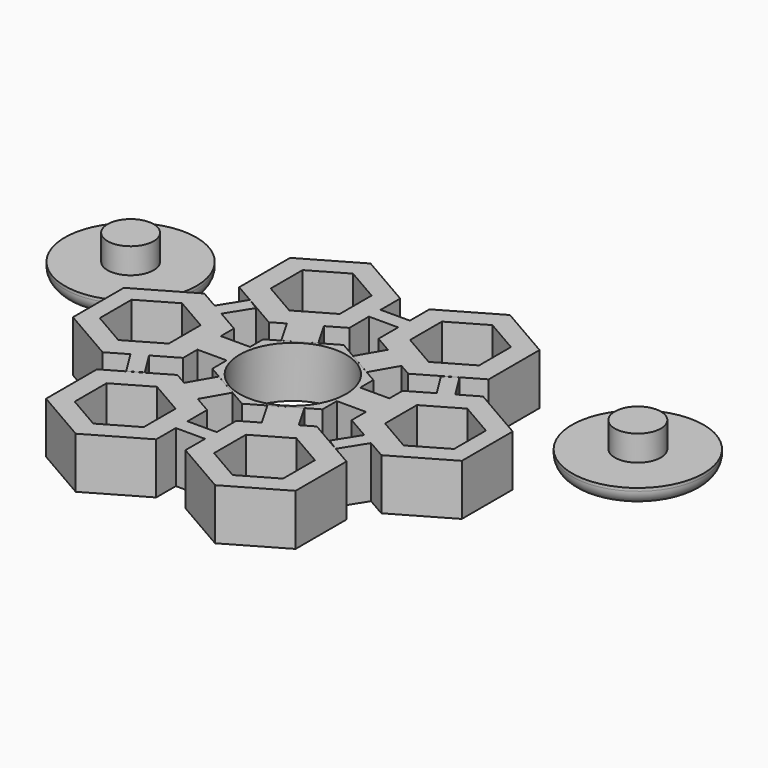
from build123d import *

# Parameters (mm, degrees)
F0_R          = 9.2578738012
F0_W          = 5.08
F0_H          = 5.08
F1_DEPTH      = 8.89
F0_H_2        = 2.54
F3_DEPTH      = 8.89
F4_R          = 11.43
F5_DEPTH      = 3.048
F6_R          = 4.0005
F7_DEPTH      = 4.445
F8_R          = 2.54
F9_TEXT_SIZE  = 11.5541534291
F10_DEPTH     = 1.524
F11_TEXT_SIZE = 11.0727295073
F12_DEPTH     = 1.524


# Not quite as in the source:
# - Text() gives the source's letters only with a copy of the font that has no kerning and outlines rounded to 1/6400 em; it was checked with that copy


with BuildPart() as f1:
    # F0 (on Top) → F1 (new body)
    with BuildSketch(Plane.XY):
        Polygon((0, -11.049), (9.5687146864, -5.5245), (9.5687146864, -2.4116488639), (9.5687146864, 2.6683511361), (9.5687146864, 5.5245), (0, 11.049), (-9.5687146864, 5.5245), (-9.5687146864, 2.6683511361), (-9.5687146864, -2.4116488639), (-9.5687146864, -5.5245), align=None)
        Circle(F0_R, mode=Mode.SUBTRACT)
        with Locations((12.1087146864, 0.1283511361)):
            Rectangle(F0_W, F0_H)
        Polygon((14.6487146864, 2.6683511361), (14.6487146864, -2.4116488639), (14.6487146864, -5.5245), (18.7068587437, -7.8674705639), (18.755828354, -7.7893427723), (20.908012187, -9.1383070969), (24.2174293728, -11.049), (33.7861440592, -5.5245), (33.7861440592, 5.5245), (24.2174293728, 11.049), (20.908012187, 9.1383070969), (18.755828354, 7.7893427723), (18.7068587437, 7.8674705639), (14.6487146864, 5.5245), align=None)
        with Locations((-12.1087146864, 0.1283511361)):
            Rectangle(F0_W, F0_H)
        Polygon((-14.6487146864, -5.5245), (-14.6487146864, -2.4116488639), (-14.6487146864, 2.6683511361), (-14.6487146864, 5.5245), (-18.7068587437, 7.8674705639), (-18.755828354, 7.7893427723), (-20.908012187, 9.1383070969), (-24.2174293728, 11.049), (-33.7861440592, 5.5245), (-33.7861440592, -5.5245), (-24.2174293728, -11.049), (-20.908012187, -9.1383070969), (-18.755828354, -7.7893427723), (-18.7068587437, -7.8674705639), align=None)
        Polygon((18.755828354, -7.7893427723), (18.7068587437, -7.8674705639), (20.908012187, -9.1383070969), align=None)
        Polygon((20.908012187, -9.1383070969), (18.7068587437, -7.8674705639), (16.0578997049, -12.0937104384), (18.2100835379, -13.4426747629), align=None)
        Polygon((16.0578997049, 12.0937104384), (18.7068587437, 7.8674705639), (20.908012187, 9.1383070969), (18.2100835379, 13.4426747629), align=None)
        Polygon((20.908012187, 9.1383070969), (18.7068587437, 7.8674705639), (18.755828354, 7.7893427723), align=None)
        Polygon((-16.0578997049, -12.0937104384), (-18.7068587437, -7.8674705639), (-20.908012187, -9.1383070969), (-18.2100835379, -13.4426747629), align=None)
        Polygon((-20.908012187, -9.1383070969), (-18.7068587437, -7.8674705639), (-18.755828354, -7.7893427723), align=None)
        Polygon((-18.755828354, 7.7893427723), (-18.7068587437, 7.8674705639), (-20.908012187, 9.1383070969), align=None)
        Polygon((-20.908012187, 9.1383070969), (-18.7068587437, 7.8674705639), (-16.0578997049, 12.0937104384), (-18.2100835379, 13.4426747629), align=None)
    extrude(amount=F1_DEPTH)


with BuildPart() as f1b:
    # F0 (on Top) → F1, piece 2 (new body)
    with BuildSketch(Plane.XY):
        Polygon((-2.54, 22.2429095143), (-2.54, 26.4974090512), (-12.1087146864, 32.0219090512), (-21.6774293728, 26.4974090512), (-21.6774293728, 15.4484090512), (-12.1087146864, 9.9239090512), (-9.9598295231, 11.1645684787), (-9.9618139168, 11.1680055493), (-5.5624048655, 13.7080055493), (-5.5604204719, 13.7045684787), (-2.54, 15.4484090512), (-2.54, 19.7029095143), align=None)
        with Locations((0, 20.9729095143)):
            Rectangle(F0_W, F0_H_2)
        Polygon((2.54, 26.4974090512), (2.54, 22.2429095143), (2.54, 19.7029095143), (2.54, 15.4484090512), (5.5604204719, 13.7045684787), (5.5624048655, 13.7080055493), (9.9618139168, 11.1680055493), (9.9598295231, 11.1645684787), (12.1087146864, 9.9239090512), (21.6774293728, 15.4484090512), (21.6774293728, 26.4974090512), (12.1087146864, 32.0219090512), align=None)
        Polygon((-3.0224048655, 9.3085964981), (-5.5604204719, 13.7045684787), (-9.9598295231, 11.1645684787), (-7.4218139168, 6.7685964981), align=None)
        Polygon((-9.9598295231, 11.1645684787), (-5.5604204719, 13.7045684787), (-5.5624048655, 13.7080055493), (-9.9618139168, 11.1680055493), align=None)
        Polygon((5.5624048655, 13.7080055493), (5.5604204719, 13.7045684787), (9.9598295231, 11.1645684787), (9.9618139168, 11.1680055493), align=None)
        Polygon((9.9598295231, 11.1645684787), (5.5604204719, 13.7045684787), (3.0224048655, 9.3085964981), (7.4218139168, 6.7685964981), align=None)
    extrude(amount=F1_DEPTH)


with BuildPart() as f1c:
    # F0 (on Top) → F1, piece 3 (new body)
    with BuildSketch(Plane.XY):
        Polygon((-12.1087146864, -32.0219090512), (-2.54, -26.4974090512), (-2.54, -22.2429095143), (-2.54, -19.7029095143), (-2.54, -15.4484090512), (-5.5604204719, -13.7045684787), (-5.5624048655, -13.7080055493), (-9.9618139168, -11.1680055493), (-9.9598295231, -11.1645684787), (-12.1087146864, -9.9239090512), (-21.6774293728, -15.4484090512), (-21.6774293728, -26.4974090512), align=None)
        with Locations((0, -20.9729095143)):
            Rectangle(F0_W, F0_H_2)
        Polygon((2.54, -19.7029095143), (2.54, -22.2429095143), (2.54, -26.4974090512), (12.1087146864, -32.0219090512), (21.6774293728, -26.4974090512), (21.6774293728, -15.4484090512), (12.1087146864, -9.9239090512), (9.9598295231, -11.1645684787), (9.9618139168, -11.1680055493), (5.5624048655, -13.7080055493), (5.5604204719, -13.7045684787), (2.54, -15.4484090512), align=None)
        Polygon((-5.5624048655, -13.7080055493), (-5.5604204719, -13.7045684787), (-9.9598295231, -11.1645684787), (-9.9618139168, -11.1680055493), align=None)
        Polygon((-9.9598295231, -11.1645684787), (-5.5604204719, -13.7045684787), (-3.0224048655, -9.3085964981), (-7.4218139168, -6.7685964981), align=None)
        Polygon((3.0224048655, -9.3085964981), (5.5604204719, -13.7045684787), (9.9598295231, -11.1645684787), (7.4218139168, -6.7685964981), align=None)
        Polygon((9.9598295231, -11.1645684787), (5.5604204719, -13.7045684787), (5.5624048655, -13.7080055493), (9.9618139168, -11.1680055493), align=None)
    extrude(amount=F1_DEPTH)


with BuildPart() as f3_tool:
    # F2 (on face) → F3 (new body)
    with BuildSketch(Plane(origin=(0, 0, 0), x_dir=(1, 0, 0), z_dir=(0, 0, -1))):
        Polygon((-6.1145198541, 17.8283906758), (-6.1145198541, 24.7498906758), (-12.1087146864, 28.2106406758), (-18.1029095187, 24.7498906758), (-18.1029095187, 17.8283906758), (-12.1087146864, 14.3676406758), align=None)
        Polygon((18.1029095187, 17.8283906758), (18.1029095187, 24.7498906758), (12.1087146864, 28.2106406758), (6.1145198541, 24.7498906758), (6.1145198541, 17.8283906758), (12.1087146864, 14.3676406758), align=None)
        Polygon((30.7817236674, 3.4613723855), (24.7864508319, 6.922744771), (18.7911779963, 3.4613723855), (18.7911779963, -3.4613723855), (24.7864508319, -6.922744771), (30.7817236674, -3.4613723855), align=None)
        Polygon((-18.7911779963, -3.4613723855), (-18.7911779963, 3.4613723855), (-24.7864508319, 6.922744771), (-30.7817236674, 3.4613723855), (-30.7817236674, -3.4613723855), (-24.7864508319, -6.922744771), align=None)
        Polygon((-6.1145198541, -17.8283906758), (-12.1087146864, -14.3676406758), (-18.1029095187, -17.8283906758), (-18.1029095187, -24.7498906758), (-12.1087146864, -28.2106406758), (-6.1145198541, -24.7498906758), align=None)
        Polygon((12.1087146864, -14.3676406758), (6.1145198541, -17.8283906758), (6.1145198541, -24.7498906758), (12.1087146864, -28.2106406758), (18.1029095187, -24.7498906758), (18.1029095187, -17.8283906758), align=None)
    extrude(amount=-F3_DEPTH)


with BuildPart() as f1_1:
    add(f1.part)

    # F3: cut by f3_tool
    add(f3_tool.part, mode=Mode.SUBTRACT)


with BuildPart() as f1b_1:
    add(f1b.part)

    # F3: cut by f3_tool
    add(f3_tool.part, mode=Mode.SUBTRACT)


with BuildPart() as f1c_1:
    add(f1c.part)

    # F3: cut by f3_tool
    add(f3_tool.part, mode=Mode.SUBTRACT)


with BuildPart() as f5:
    # F4 (on Top) → F5 (new body)
    with BuildSketch(Plane.XY):
        with Locations((43.2678200305, 20.853670314)):
            Circle(F4_R)
    extrude(amount=F5_DEPTH)

    # F6 (on face) → F7 (join)
    with BuildSketch(Plane.XY.offset(3.048)):
        with Locations((43.2678200305, 20.853670314)):
            Circle(F6_R)
    extrude(amount=F7_DEPTH)

    # F8
    f8_edges = [f5.edges().sort_by_distance(p)[0] for p in [
        (31.83782, 20.85367, 0),
    ]]
    fillet(f8_edges, radius=F8_R)

    # F9 (on face) → F10 (cut)
    with BuildSketch(Plane(origin=(0, 0, 0), x_dir=(1, 0, 0), z_dir=(0, 0, -1))):
        with Locations((43.0414924987, -25.1126140356)):
            Text('B', F9_TEXT_SIZE, font='Open Sans', font_style=FontStyle.ITALIC, text_align=(TextAlign.LEFT, TextAlign.BOTTOM))
    extrude(amount=-F10_DEPTH, mode=Mode.SUBTRACT)

    # F11 (on face) → F12 (cut)
    with BuildSketch(Plane(origin=(0, 0, 0), x_dir=(1, 0, 0), z_dir=(0, 0, -1))):
        with Locations((35.9684824944, -25.0259581953)):
            Text('D', F11_TEXT_SIZE, font='Open Sans', font_style=FontStyle.ITALIC, text_align=(TextAlign.LEFT, TextAlign.BOTTOM))
    extrude(amount=-F12_DEPTH, mode=Mode.SUBTRACT)


with BuildPart() as f13_1:
    # F13: copy of F5
    add(f5.part.moved(Location((-88.138, 0, 0))))


solid = Compound([f1_1.part, f1b_1.part, f1c_1.part, f5.part, f13_1.part])
